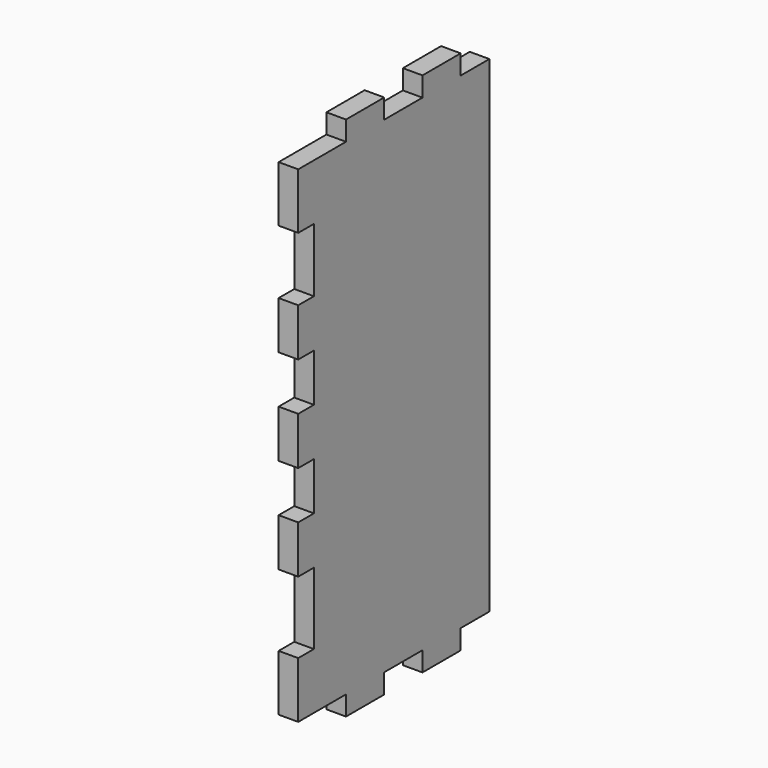
from build123d import *

# Parameters (mm, degrees)
F0_W     = 63.5
F0_H     = 139.7
F1_DEPTH = 5.207
F2_W     = 5.207
F2_H     = 16.9333164
F2_H_2   = 12.7
F2_H_3   = 19.05
F2_W_2   = 15.875
F2_H_4   = 5.207
F2_W_3   = 12.7
F2_W_4   = 9.525
F3_DEPTH = 5.208


# Not quite as in the source:
# - a feature names something its author has since deleted; it is built from what else it names


with BuildPart() as f1:
    # F0 (on Right) → F1 (new body)
    with BuildSketch(Plane.YZ):
        Rectangle(F0_W, F0_H)
    extrude(amount=F1_DEPTH)

    # F2 (on face) → F3 (cut, through all)
    with BuildSketch(Plane.YZ.offset(5.207)):
        with Locations((-29.1465, 41.3046418)):
            Rectangle(F2_W, F2_H)
        with Locations((-29.1465, 13.7879836)):
            Rectangle(F2_W, F2_H_2)
        with Locations((-29.1465, -11.6120164)):
            Rectangle(F2_W, F2_H_2)
        with Locations((-29.1465, -40.1870164)):
            Rectangle(F2_W, F2_H_3)
        with Locations((-23.8125, -67.2465)):
            Rectangle(F2_W_2, F2_H_4)
        with Locations((3.175, -67.2465)):
            Rectangle(F2_W_3, F2_H_4)
        with Locations((26.9875, -67.2465)):
            Rectangle(F2_W_4, F2_H_4)
        with Locations((26.9875, 67.2465)):
            Rectangle(F2_W_4, F2_H_4)
        with Locations((3.175, 67.2465)):
            Rectangle(F2_W_3, F2_H_4)
        with Locations((-23.8125, 67.2465)):
            Rectangle(F2_W_2, F2_H_4)
    extrude(amount=-F3_DEPTH, mode=Mode.SUBTRACT)


solid = f1.part
